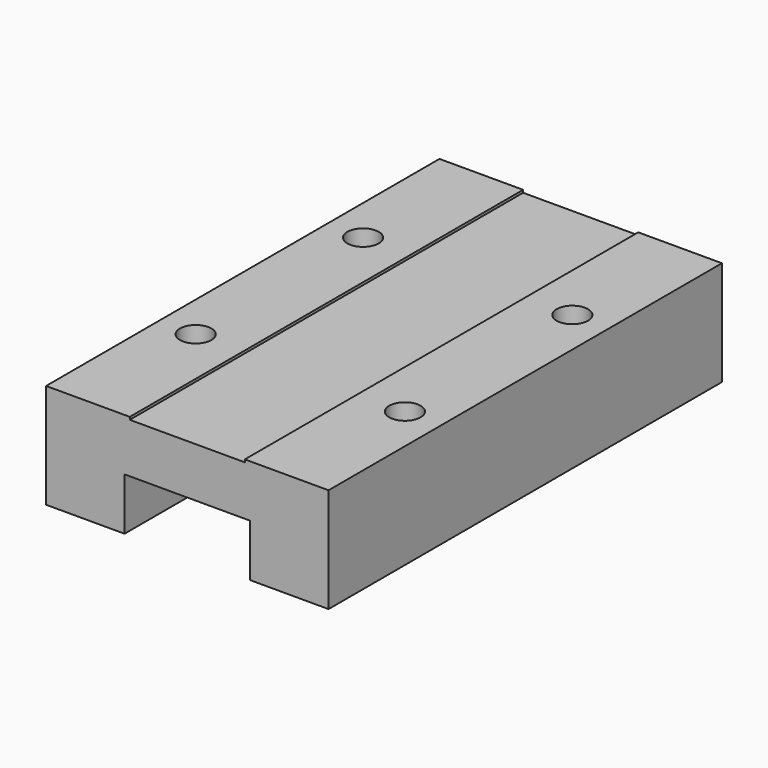
from build123d import *

# Parameters (mm, degrees)
F1_DEPTH = 23.5
F3_D     = 3
F3_DEPTH = 4
F3_TIP   = 0.9012909285


with BuildPart() as f1:
    # F0 (on Front) → F1 (new body, symmetric)
    with BuildSketch(Plane.XZ):
        Polygon((-5.5, 5), (-13.5, 5), (-13.5, -5), (-6, -5), (-6, 0), (6, 0), (6, -5), (13.5, -5), (13.5, 5), (5.5, 5), (5.5, 4.75), (-5.5, 4.75), align=None)
    extrude(amount=F1_DEPTH, both=True)

    # F3
    with Locations(Plane.XY.offset(5)):
        with Locations((-10.0000007078, 10), (10.0000007078, 10), (10.0000007078, -10), (-10.0000007078, -10)):
            Hole(F3_D / 2, depth=F3_DEPTH)
            with Locations((0, 0, -(F3_DEPTH + F3_TIP / 2))):  # 118° drill point
                Cone(0, F3_D / 2, F3_TIP, mode=Mode.SUBTRACT)


solid = f1.part
